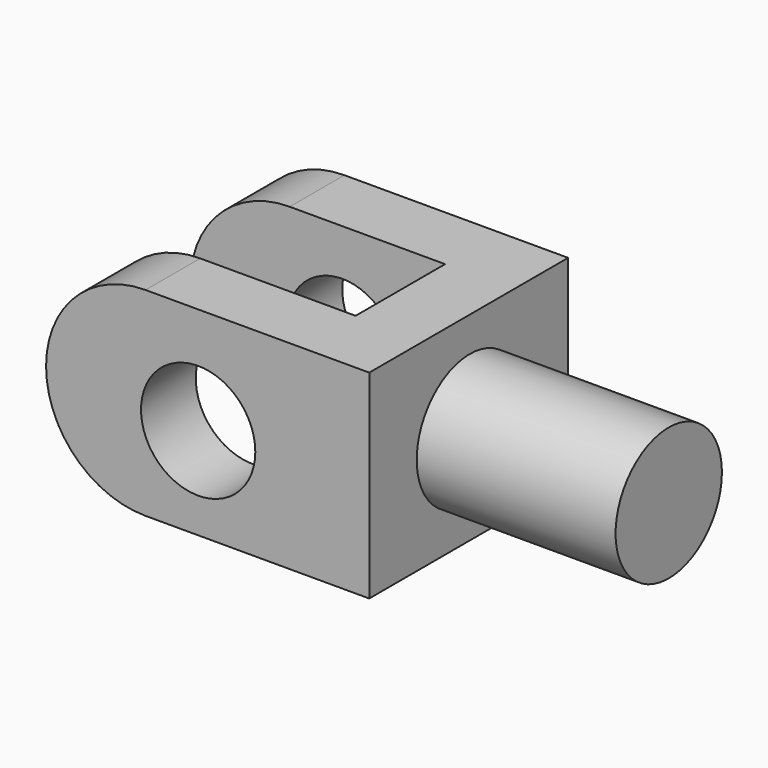
from build123d import *

# Parameters (mm, degrees)
F1_DEPTH  = 32
F2_R      = 9.193205317
F4_DEPTH  = 11
F3_R      = 8.8221237906
F5_DEPTH  = 50.8
F6_R      = 16
F7_R      = 15.99999
F8_R      = 16
F9_R      = 15.99999
F10_R     = 10.6938119657
F11_DEPTH = 32


# Not quite as in the source:
# - a fillet or chamfer is up to 0.001 mm smaller than in the source, because OpenCascade refuses the exact size


with BuildPart() as f1:
    # F0 (on Top) → F1 (new body)
    with BuildSketch(Plane.XY):
        Polygon((16.5285665829, 19.762864985), (-24.4714334171, 19.762864985), (-24.4714334171, 8.762864985), (16.5285665829, 8.762864985), (16.5285665829, -9.237135015), (-24.4714334171, -9.237135015), (-24.4714334171, -20.237135015), (27.5285665829, -20.237135015), (27.5285665829, 19.762864985), align=None)
    extrude(amount=F1_DEPTH)

    # F2 (on face) → F4 (cut)
    with BuildSketch(Plane.XZ.offset(20.237135015)):
        with Locations((0, 14.8110119626)):
            Circle(F2_R)
    extrude(amount=-F4_DEPTH, mode=Mode.SUBTRACT)

    # F3 (on Front) → F5 (cut)
    with BuildSketch(Plane.XZ):
        with Locations((0, 15.7271567732)):
            Circle(F3_R)
    extrude(amount=-F5_DEPTH, mode=Mode.SUBTRACT)

    # F6
    f6_edges = [f1.edges().sort_by_distance(p)[0] for p in [
        (-24.471433, -14.737135, 32),
    ]]
    fillet(f6_edges, radius=F6_R)

    # F7 (radius 16 in the source; OpenCascade refuses exactly that, so slightly less here)
    f7_edges = [f1.edges().sort_by_distance(p)[0] for p in [
        (-24.471433, -14.737135, 0),
    ]]
    fillet(f7_edges, radius=F7_R)

    # F8
    f8_edges = [f1.edges().sort_by_distance(p)[0] for p in [
        (-24.471433, 14.262865, 32),
    ]]
    fillet(f8_edges, radius=F8_R)

    # F9 (radius 16 in the source; OpenCascade refuses exactly that, so slightly less here)
    f9_edges = [f1.edges().sort_by_distance(p)[0] for p in [
        (-24.471433, 14.262865, 0),
    ]]
    fillet(f9_edges, radius=F9_R)

    # F10 (on face) → F11 (join)
    with BuildSketch(Plane.YZ.offset(27.5285665829)):
        with Locations((0, 15.7271567732)):
            Circle(F10_R)
    extrude(amount=F11_DEPTH)


solid = f1.part
